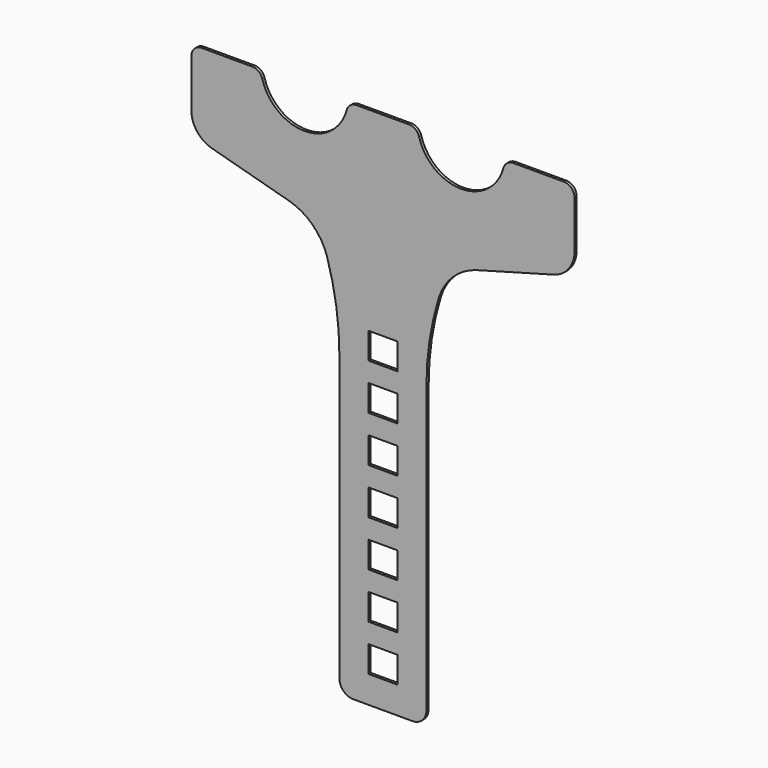
from build123d import *

# Parameters (mm, degrees)
F0_W        = 10.4902
F0_H        = 9.6012
F1_DEPTH    = 1.00584
F2_R        = 20.32
F3_R        = 10.16
F4_R        = 3.81
F5_R        = 3.81
F6_T1_DEPTH = 1.00584
F7_R        = 5.08


# Not quite as in the source:
# - a fillet or chamfer that OpenCascade refuses, or shapes differently, is made with other operations: its cross-section is extruded or revolved along the edge and cut away or added


with BuildPart() as f1:
    # F0 (on Front) → F1 (new body)
    with BuildSketch(Plane.XZ):
        with BuildLine():
            Line((-44.45, 0), (-69.85, 0))
            Line((-69.85, 0), (-69.85, -28.956))
            Line((-69.85, -28.956), (-23.7198378891, -41.5853487635))
            Line((-23.7198378891, -41.5853487635), (-15.875, -66.2231149459))
            Line((-15.875, -66.2231149459), (-15.875, -191.0842))
            Line((-15.875, -191.0842), (0, -191.0842))
            Line((0, -191.0842), (15.875, -191.0842))
            Line((15.875, -191.0842), (15.875, -66.2231149459))
            Line((15.875, -66.2231149459), (23.7198378891, -41.5853487635))
            Line((23.7198378891, -41.5853487635), (69.85, -28.956))
            Line((69.85, -28.956), (69.85, 0))
            Line((69.85, 0), (44.45, 0))
            ThreePointArc((44.45, 0), (28.575, -14.478), (12.7, 0))
            Line((12.7, 0), (-12.7, 0))
            ThreePointArc((-12.7, 0), (-28.575, -14.478), (-44.45, 0))
        make_face()
        with Locations((0, -176.3776)):
            Rectangle(F0_W, F0_H, mode=Mode.SUBTRACT)
        with Locations((0, -159.6136)):
            Rectangle(F0_W, F0_H, mode=Mode.SUBTRACT)
        with Locations((0, -142.8496)):
            Rectangle(F0_W, F0_H, mode=Mode.SUBTRACT)
        with Locations((0, -126.0856)):
            Rectangle(F0_W, F0_H, mode=Mode.SUBTRACT)
        with Locations((0, -109.3216)):
            Rectangle(F0_W, F0_H, mode=Mode.SUBTRACT)
        with Locations((0, -92.5576)):
            Rectangle(F0_W, F0_H, mode=Mode.SUBTRACT)
        with Locations((0, -75.7936)):
            Rectangle(F0_W, F0_H, mode=Mode.SUBTRACT)
    extrude(amount=-F1_DEPTH)

    # F2
    f2_edges = [f1.edges().sort_by_distance(p)[0] for p in [
        (-23.719838, 0.50292, -41.585349),
        (23.719838, 0.50292, -41.585349),
    ]]
    fillet(f2_edges, radius=F2_R)

    # F3
    f3_edges = [f1.edges().sort_by_distance(p)[0] for p in [
        (-69.85, 0.50292, -28.956),
        (69.85, 0.50292, -28.956),
    ]]
    fillet(f3_edges, radius=F3_R)

    # F4
    f4_edges = [f1.edges().sort_by_distance(p)[0] for p in [
        (69.85, 0.50292, 0),
        (-69.85, 0.50292, 0),
    ]]
    fillet(f4_edges, radius=F4_R)

    # F5
    f5_edges = [f1.edges().sort_by_distance(p)[0] for p in [
        (44.45, 0.50292, 0),
        (-44.45, 0.50292, 0),
        (-12.7, 0.50292, 0),
        (12.7, 0.50292, 0),
    ]]
    fillet(f5_edges, radius=F5_R)

    # F6: fillet of radius 101.6 on 2 edges, made by hand

    # F6_s2 → F6_t1 (join)
    with BuildSketch(Plane.XZ.offset(-1.00584)):
        with BuildLine():
            ThreePointArc((15.875, -81.9921288589), (17.0051850195, -66.880005322), (20.3705960196, -52.1040923291))
            Line((20.3705960196, -52.1040923291), (18.42850794, -51.5063315985))
            ThreePointArc((18.42850794, -51.5063315985), (16.1865788547, -58.5470978522), (13.9387808449, -65.6066091605))
            Line((13.9387808449, -65.6066091605), (13.843, -66.2231149459))
            Line((13.843, -66.2231149459), (13.843, -81.9921288589))
            Line((13.843, -81.9921288589), (15.875, -81.9921288589))
        make_face()
        with BuildLine():
            ThreePointArc((-20.3705960196, -52.1040923291), (-17.0051850195, -66.880005322), (-15.875, -81.9921288589))
            Line((-15.875, -81.9921288589), (-13.843, -81.9921288589))
            Line((-13.843, -81.9921288589), (-13.843, -66.2231149459))
            Line((-13.843, -66.2231149459), (-13.9387808449, -65.6066091605))
            ThreePointArc((-13.9387808449, -65.6066091605), (-16.1865788547, -58.5470978522), (-18.42850794, -51.5063315985))
            Line((-18.42850794, -51.5063315985), (-20.3705960196, -52.1040923291))
        make_face()
    extrude(amount=F6_T1_DEPTH)

    # F7
    f7_edges = [f1.edges().sort_by_distance(p)[0] for p in [
        (15.875, 0.50292, -191.0842),
        (-15.875, 0.50292, -191.0842),
    ]]
    fillet(f7_edges, radius=F7_R)


solid = f1.part
